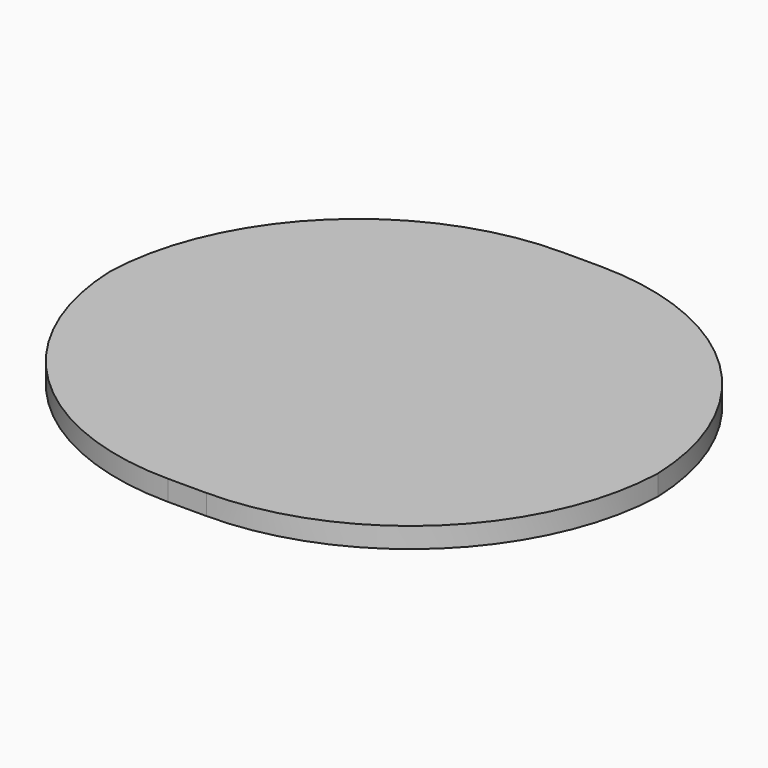
from build123d import *

# Parameters (mm, degrees)
F0_W        = 268.8191002235
F0_H        = 241.1657162011
F1_DEPTH    = 10
F2_T1_DEPTH = 635


# Not quite as in the source:
# - a fillet or chamfer that OpenCascade refuses, or shapes differently, is made with other operations: its cross-section is extruded or revolved along the edge and cut away or added


with BuildPart() as f1:
    # F0 (on Top) → F1 (new body)
    with BuildSketch(Plane.XY):
        with Locations((-4.3010744266, 5.1392484456)):
            Rectangle(F0_W, F0_H)
    extrude(amount=F1_DEPTH)

    # F2: fillet of radius 125 on 4 edges, made by hand

    # F2_s2 → F2_t1 (cut)
    with BuildSketch(Plane.XY.offset(-312.5)):
        with BuildLine():
            ThreePointArc((-13.7106245384, -115.4436096549), (-102.0989721867, -78.8319573032), (-138.7106245384, 9.5563903451))
            Line((-138.7106245384, 9.5563903451), (-138.7106245384, -115.4436096549))
            Line((-138.7106245384, -115.4436096549), (-13.7106245384, -115.4436096549))
        make_face()
        with BuildLine():
            ThreePointArc((5.1084756851, -115.4436096549), (93.4968233334, -78.8319573032), (130.1084756851, 9.5563903451))
            Line((130.1084756851, 9.5563903451), (130.1084756851, -115.4436096549))
            Line((130.1084756851, -115.4436096549), (5.1084756851, -115.4436096549))
        make_face()
        with BuildLine():
            ThreePointArc((130.1084756851, 0.7221065462), (93.4968233334, 89.1104541945), (5.1084756851, 125.7221065462))
            Line((5.1084756851, 125.7221065462), (130.1084756851, 125.7221065462))
            Line((130.1084756851, 125.7221065462), (130.1084756851, 0.7221065462))
        make_face()
        with BuildLine():
            ThreePointArc((-13.7106245384, 125.7221065462), (-102.0989721867, 89.1104541945), (-138.7106245384, 0.7221065462))
            Line((-138.7106245384, 0.7221065462), (-138.7106245384, 125.7221065462))
            Line((-138.7106245384, 125.7221065462), (-13.7106245384, 125.7221065462))
        make_face()
    extrude(amount=F2_T1_DEPTH, mode=Mode.SUBTRACT)


solid = f1.part
